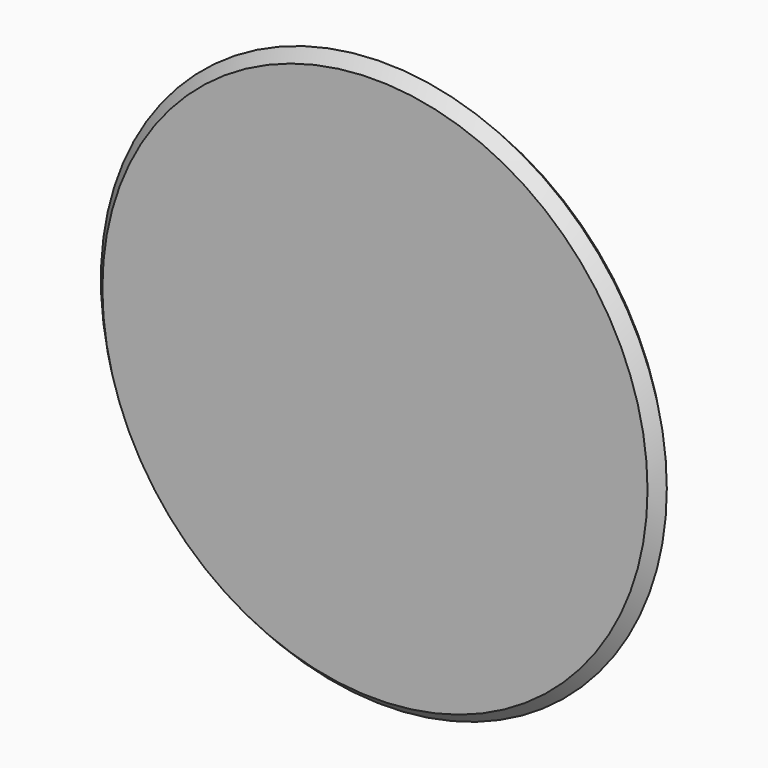
from build123d import *

# Parameters (mm, degrees)
F0_R     = 127
F0_R_2   = 5
F1_DEPTH = 5
F2_DEPTH = 5
F3_SIZE2 = 4.662565
F3_SIZE  = 4.99999


# Not quite as in the source:
# - a fillet or chamfer is up to 0.001 mm smaller than in the source, because OpenCascade refuses the exact size


with BuildPart() as f1:
    # F0 (on Front) → F1 (new body, symmetric)
    with BuildSketch(Plane.XZ):
        Circle(F0_R)
        Circle(F0_R_2, mode=Mode.SUBTRACT)
    extrude(amount=F1_DEPTH, both=True)

    # F0 (on Front) → F2 (join, symmetric)
    with BuildSketch(Plane.XZ):
        Circle(F0_R_2)
    extrude(amount=F2_DEPTH, both=True)

    # F3 (size 5 and 4.6625754307 in the source; OpenCascade refuses exactly that, so slightly less here)
    f3_edges = [f1.edges().sort_by_distance(p)[0] for p in [
        (-127, 5, 0),
        (-127, -5, 0),
    ]]
    f3_side = f1.faces().sort_by_distance((-127, 0, 0))[0]
    chamfer(f3_edges, length=F3_SIZE, length2=F3_SIZE2, reference=f3_side)


solid = f1.part
